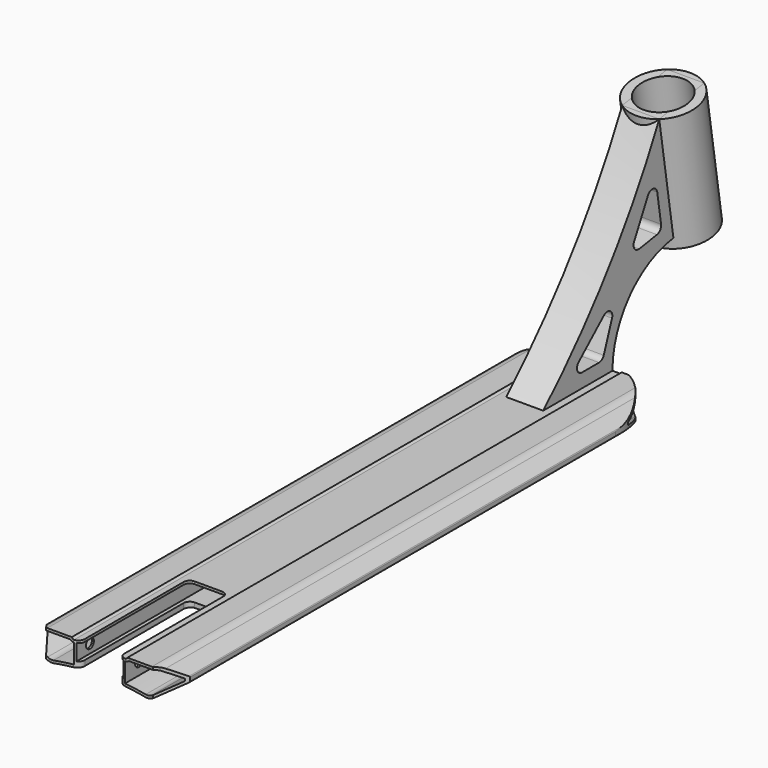
from build123d import *

# Parameters (mm, degrees)
F1_DEPTH       = 250
F2_W           = 38
F2_H           = 13
F3_DEPTH       = 250
F4_T1_DEPTH    = 500
F5_R           = 9
F6_R           = 1
F8_DEPTH       = 505
F10_DEPTH      = 118.9
F10_DEPTH_BACK = 563
F12_DEPTH      = 25
F12_DEPTH_BACK = 61.0714870032
F13_T1_DEPTH   = 2
F13_T6_DEPTH   = 32
F13_S7_R       = 200
F13_T8_DEPTH   = 18
F13_T13_DEPTH  = 32
F13_S14_R      = 200
F13_T15_DEPTH  = 18
F13_T20_DEPTH  = 64.2634824315
F13_T26_DEPTH  = 34.2634824315
F13_S27_R      = 200
F13_T28_DEPTH  = 19
F13_T32_DEPTH  = 34.2634824315
F13_S33_R      = 200
F13_T34_DEPTH  = 19
F13_T38_DEPTH  = 64.2634824315
F13_T41_DEPTH  = 62
F15_D          = 8
F15_DEPTH      = 50
F15_TIP        = 2.4034424761
F17_DEPTH      = 15
F18_R          = 27.5
F19_DEPTH      = 100
F21_D          = 40
F23_DEPTH      = 72.5010001
F24_R          = 5


# Not quite as in the source:
# - a fillet or chamfer that OpenCascade refuses, or shapes differently, is made with other operations: its cross-section is extruded or revolved along the edge and cut away or added
# - an extrude ends at something that could not be found from the text; its depth is read off the source's solid


with BuildPart() as f1:
    # F0 (on Front) → F1 (new body, symmetric)
    with BuildSketch(Plane.XZ):
        with BuildLine():
            Line((22.5, 59.7704869032), (0, 59.7704869032))
            Line((0, 59.7704869032), (-22.5, 59.7704869032))
            Line((-22.5, 59.7704869032), (-22.5, 61.0704869032))
            Line((-22.5, 61.0704869032), (-45.5824640741, 61.0704869032))
            Line((-45.5824640741, 61.0704869032), (-57.5, 51.0704869032))
            Line((-57.5, 51.0704869032), (-57.5, 47.0704869032))
            Line((-57.5, 47.0704869032), (-40.1794919243, 37.0704869032))
            ThreePointArc((-40.1794919243, 37.0704869032), (0, 41.1480317616), (40.1794919243, 37.0704869032))
            Line((40.1794919243, 37.0704869032), (57.5, 47.0704869032))
            Line((57.5, 47.0704869032), (57.5, 51.0704869032))
            Line((57.5, 51.0704869032), (45.5824640741, 61.0704869032))
            Line((45.5824640741, 61.0704869032), (22.5, 61.0704869032))
            Line((22.5, 61.0704869032), (22.5, 59.7704869032))
        make_face()
    extrude(amount=F1_DEPTH, both=True)

    # F2 (on Front) → F3 (cut, symmetric)
    with BuildSketch(Plane.XZ):
        with Locations((0, 51.2704869032)):
            Rectangle(F2_W, F2_H)
    extrude(amount=F3_DEPTH, both=True, mode=Mode.SUBTRACT)

    # F4: fillet of radius 2 on 2 edges, made by hand

    # F4_s2 → F4_t1 (join)
    with BuildSketch(Plane.XZ.offset(-250)):
        with BuildLine():
            ThreePointArc((22.5, 61.0704869032), (21.7666760256, 60.1273192307), (20.6265006005, 59.7704869032))
            Line((20.6265006005, 59.7704869032), (22.5, 59.7704869032))
            Line((22.5, 59.7704869032), (22.5, 61.0704869032))
        make_face()
        with BuildLine():
            ThreePointArc((-20.6265006005, 59.7704869032), (-21.7666760256, 60.1273192307), (-22.5, 61.0704869032))
            Line((-22.5, 61.0704869032), (-22.5, 59.7704869032))
            Line((-22.5, 59.7704869032), (-20.6265006005, 59.7704869032))
        make_face()
    extrude(amount=F4_T1_DEPTH)

    # F5
    f5_edges = [f1.edges().sort_by_distance(p)[0] for p in [
        (45.582464, 0, 61.070487),
        (-45.582464, 0, 61.070487),
        (-40.179492, 0, 37.070487),
        (40.179492, 0, 37.070487),
    ]]
    fillet(f5_edges, radius=F5_R)

    # F6
    f6_edges = [f1.edges().sort_by_distance(p)[0] for p in [
        (57.5, 0, 51.070487),
        (57.5, 0, 47.070487),
        (-57.5, 0, 51.070487),
        (-57.5, 0, 47.070487),
    ]]
    fillet(f6_edges, radius=F6_R)

    # F7 (on face) → F8 (cut)
    with BuildSketch(Plane.XZ.offset(250)):
        with BuildLine():
            ThreePointArc((20.6265006005, 42.0921719424), (28.9931861118, 41.0564987136), (37.3093701274, 39.6726168907))
            ThreePointArc((37.3093701274, 39.6726168907), (39.7790673433, 39.6518088424), (42.1022690923, 40.4900038955))
            Line((42.1022690923, 40.4900038955), (55.5, 48.2251874416))
            Line((55.5, 48.2251874416), (55.5, 50.1378715869))
            Line((55.5, 50.1378715869), (46.8062452335, 57.432798005))
            ThreePointArc((46.8062452335, 57.432798005), (44.7008729689, 58.6483352487), (42.3067319657, 59.0704869032))
            Line((42.3067319657, 59.0704869032), (23.5777715132, 59.0704869032))
            ThreePointArc((23.5777715132, 59.0704869032), (22.2389521501, 58.1098858596), (20.6265006005, 57.7704869032))
            Line((20.6265006005, 57.7704869032), (20.6265006005, 42.0921719424))
        make_face()
        with BuildLine():
            ThreePointArc((-37.3093701274, 39.6726168907), (-28.9931861118, 41.0564987136), (-20.6265006005, 42.0921719424))
            Line((-20.6265006005, 42.0921719424), (-20.6265006005, 57.7704869032))
            ThreePointArc((-20.6265006005, 57.7704869032), (-22.2389521501, 58.1098858596), (-23.5777715132, 59.0704869032))
            Line((-23.5777715132, 59.0704869032), (-42.3067319657, 59.0704869032))
            ThreePointArc((-42.3067319657, 59.0704869032), (-44.7008729689, 58.6483352487), (-46.8062452335, 57.432798005))
            Line((-46.8062452335, 57.432798005), (-55.5, 50.1378715869))
            Line((-55.5, 50.1378715869), (-55.5, 48.2251874416))
            Line((-55.5, 48.2251874416), (-42.1022690923, 40.4900038955))
            ThreePointArc((-42.1022690923, 40.4900038955), (-39.7790673433, 39.6518088424), (-37.3093701274, 39.6726168907))
        make_face()
    extrude(amount=-F8_DEPTH, mode=Mode.SUBTRACT)

    # F9 (on Top) → F10 (cut, two sides)
    with BuildSketch(Plane.XY) as f10_sk:
        with BuildLine():
            ThreePointArc((-57.5, 200), (0, 257.5), (57.5, 200))
            Line((57.5, 200), (57.5, 280))
            Line((57.5, 280), (-57.5, 280))
            Line((-57.5, 280), (-57.5, 200))
        make_face()
    extrude(amount=F10_DEPTH, mode=Mode.SUBTRACT)
    extrude(f10_sk.sketch, amount=-F10_DEPTH_BACK, mode=Mode.SUBTRACT)

    # F11 (on Top) → F12 (cut, two sides)
    with BuildSketch(Plane.XY) as f12_sk:
        Polygon((-68, -346), (68, -346), (68, -216), (43.2975540478, -250), (16, -250), (16, -140), (-16, -140), (-16, -250), (-43.2975540478, -250), (-68, -216), align=None)
    extrude(amount=-F12_DEPTH, mode=Mode.SUBTRACT)
    extrude(f12_sk.sketch, amount=F12_DEPTH_BACK, mode=Mode.SUBTRACT)

    # F13: fillet of radius 5 on 6 edges, made by hand

    # F13_s2 → F13_t1 (join)
    with BuildSketch(Plane.XY.offset(57.7704869032)):
        with BuildLine():
            ThreePointArc((-11, -140), (-14.5355339059, -141.4644660941), (-16, -145))
            Line((-16, -145), (-16.1, -145))
            Line((-16.1, -145), (-16.1, -139.9))
            Line((-16.1, -139.9), (-11, -139.9))
            Line((-11, -139.9), (-11, -140))
        make_face()
        with BuildLine():
            ThreePointArc((16, -145), (14.5355339059, -141.4644660941), (11, -140))
            Line((11, -140), (11, -139.9))
            Line((11, -139.9), (16.1, -139.9))
            Line((16.1, -139.9), (16.1, -145))
            Line((16.1, -145), (16, -145))
        make_face()
    extrude(amount=F13_T1_DEPTH)


with BuildPart() as f13_tool4:
    # F13_s5 → F13_t6 (new body)
    with BuildSketch(Plane.XY.offset(59.7704869032)):
        with BuildLine():
            ThreePointArc((-11, -140), (-14.5355339059, -141.4644660941), (-16, -145))
            Line((-16, -145), (-16.1, -145))
            Line((-16.1, -145), (-16.1, -139.9))
            Line((-16.1, -139.9), (-11, -139.9))
            Line((-11, -139.9), (-11, -140))
        make_face()
    extrude(amount=-F13_T6_DEPTH)

    # F13_s7 → F13_t8 (cut, symmetric)
    with BuildSketch(Plane.XZ.offset(142.4)):
        with Locations((0, -158.8519682384)):
            Circle(F13_S7_R)
    extrude(amount=F13_T8_DEPTH, both=True, mode=Mode.SUBTRACT)

    split(bisect_by=Plane.XY.offset(44.7704869032), keep=Keep.BOTTOM)


with BuildPart() as f1_1:
    add(f1.part)

    # F13_t3: union F13_tool4
    add(f13_tool4.part)


with BuildPart() as f13_tool11:
    # F13_s12 → F13_t13 (new body)
    with BuildSketch(Plane.XY.offset(27.7704869032)):
        with BuildLine():
            ThreePointArc((16, -145), (14.5355339059, -141.4644660941), (11, -140))
            Line((11, -140), (11, -139.9))
            Line((11, -139.9), (16.1, -139.9))
            Line((16.1, -139.9), (16.1, -145))
            Line((16.1, -145), (16, -145))
        make_face()
    extrude(amount=F13_T13_DEPTH)

    # F13_s14 → F13_t15 (cut, symmetric)
    with BuildSketch(Plane.XZ.offset(142.4)):
        with Locations((0, -158.8519682384)):
            Circle(F13_S14_R)
    extrude(amount=F13_T15_DEPTH, both=True, mode=Mode.SUBTRACT)

    split(bisect_by=Plane.XY.offset(44.7704869032), keep=Keep.BOTTOM)


with BuildPart() as f1_2:
    add(f1_1.part)

    # F13_t10: union F13_tool11
    add(f13_tool11.part)


with BuildPart() as f13_tool18:
    # F13_s19 → F13_t20 (new body)
    with BuildSketch(Plane.XY.offset(74.7704869032)):
        with BuildLine():
            ThreePointArc((-16, -145), (-14.5355339059, -141.4644660941), (-11, -140))
            Line((-11, -140), (-11, -139.9))
            Line((-11, -139.9), (-16.1, -139.9))
            Line((-16.1, -139.9), (-16.1, -145))
            Line((-16.1, -145), (-16, -145))
        make_face()
    extrude(amount=-F13_T20_DEPTH)

    split(bisect_by=Plane.XY.offset(57.7704869032), keep=Keep.TOP)

    split(bisect_by=Plane.XY.offset(59.7704869032), keep=Keep.BOTTOM)


with BuildPart() as f1_3:
    add(f1_2.part)

    # F13_t17: union F13_tool18
    add(f13_tool18.part)


with BuildPart() as f13_tool24:
    # F13_s25 → F13_t26 (new body)
    with BuildSketch(Plane.XY.offset(44.7704869032)):
        with BuildLine():
            ThreePointArc((-16, -145), (-14.5355339059, -141.4644660941), (-11, -140))
            Line((-11, -140), (-11, -139.9))
            Line((-11, -139.9), (-16.1, -139.9))
            Line((-16.1, -139.9), (-16.1, -145))
            Line((-16.1, -145), (-16, -145))
        make_face()
    extrude(amount=-F13_T26_DEPTH)

    # F13_s27 → F13_t28 (cut, symmetric)
    with BuildSketch(Plane.XZ.offset(142.4)):
        with Locations((0, -158.8519682384)):
            Circle(F13_S27_R)
    extrude(amount=F13_T28_DEPTH, both=True, mode=Mode.SUBTRACT)


with BuildPart() as f1_4:
    add(f1_3.part)

    # F13_t23: union F13_tool24
    add(f13_tool24.part)


with BuildPart() as f13_tool30:
    # F13_s31 → F13_t32 (new body)
    with BuildSketch(Plane.XY.offset(10.5070044716)):
        with BuildLine():
            ThreePointArc((16, -145), (14.5355339059, -141.4644660941), (11, -140))
            Line((11, -140), (11, -139.9))
            Line((11, -139.9), (16.1, -139.9))
            Line((16.1, -139.9), (16.1, -145))
            Line((16.1, -145), (16, -145))
        make_face()
    extrude(amount=F13_T32_DEPTH)

    # F13_s33 → F13_t34 (cut, symmetric)
    with BuildSketch(Plane.XZ.offset(142.4)):
        with Locations((0, -158.8519682384)):
            Circle(F13_S33_R)
    extrude(amount=F13_T34_DEPTH, both=True, mode=Mode.SUBTRACT)


with BuildPart() as f1_5:
    add(f1_4.part)

    # F13_t29: union F13_tool30
    add(f13_tool30.part)


with BuildPart() as f13_tool36:
    # F13_s37 → F13_t38 (new body)
    with BuildSketch(Plane.XY.offset(10.5070044716)):
        with BuildLine():
            ThreePointArc((16, -145), (14.5355339059, -141.4644660941), (11, -140))
            Line((11, -140), (11, -139.9))
            Line((11, -139.9), (16.1, -139.9))
            Line((16.1, -139.9), (16.1, -145))
            Line((16.1, -145), (16, -145))
        make_face()
    extrude(amount=F13_T38_DEPTH)

    split(bisect_by=Plane.XY.offset(57.7704869032), keep=Keep.TOP)

    split(bisect_by=Plane.XY.offset(59.7704869032), keep=Keep.BOTTOM)


with BuildPart() as f1_6:
    add(f1_5.part)

    # F13_t35: union F13_tool36
    add(f13_tool36.part)

    # F13_s42 → F13_t41 (cut)
    with BuildSketch(Plane.XY.offset(27.7704869032)):
        with BuildLine():
            ThreePointArc((-21, -250), (-17.4644660941, -248.5355339059), (-16, -245))
            Line((-16, -245), (-15.9, -245))
            Line((-15.9, -245), (-15.9, -250.1))
            Line((-15.9, -250.1), (-21, -250.1))
            Line((-21, -250.1), (-21, -250))
        make_face()
        with BuildLine():
            ThreePointArc((21, -250), (17.4644660941, -248.5355339059), (16, -245))
            Line((16, -245), (15.9, -245))
            Line((15.9, -245), (15.9, -250.1))
            Line((15.9, -250.1), (21, -250.1))
            Line((21, -250.1), (21, -250))
        make_face()
    extrude(amount=F13_T41_DEPTH, mode=Mode.SUBTRACT)

    # F15 (one way)
    with BuildSketch(Plane.YZ.offset(20.6265006005)):
        with Locations((-235.9860303046, 52.0921719424)):
            Circle(F15_D / 2)
    extrude(amount=-F15_DEPTH, mode=Mode.SUBTRACT)
    with Locations(Plane.YZ.offset(20.6265006005)):
        with Locations((-235.9860303046, 52.0921719424)):
            with Locations((0, 0, -(F15_DEPTH + F15_TIP / 2))):  # 118° drill point
                Cone(0, F15_D / 2, F15_TIP, mode=Mode.SUBTRACT)

    # F16 (on Right) → F17 (join, symmetric)
    with BuildSketch(Plane.YZ):
        with BuildLine():
            ThreePointArc((297.3819995028, 219.7704869032), (245.9666940414, 134.4327647562), (180, 59.7704869032))
            Line((180, 59.7704869032), (250, 59.7704869032))
            ThreePointArc((250, 59.7704869032), (267.6550746197, 106.2463815899), (311.7145367693, 129.2784080277))
            Line((311.7145367693, 129.2784080277), (313.0254460068, 121.0016528437))
            Line((313.0254460068, 121.0016528437), (358.4591096742, 128.1976382355))
            Line((358.4591096742, 128.1976382355), (342.8156631702, 226.966472295))
            Line((342.8156631702, 226.966472295), (297.3819995028, 219.7704869032))
        make_face()
    extrude(amount=F17_DEPTH, both=True)

    # F18 (on face) → F19 (join)
    with BuildSketch(Plane(origin=(0, -26.6789521342, 168.4442744471), x_dir=(1, 0, 0), z_dir=(0, -0.156434465, 0.9876883406))):
        with Locations((0, 351.1004121621)):
            Circle(F18_R)
    extrude(amount=-F19_DEPTH)

    # F21 (through all)
    with Locations(Plane(origin=(0, -26.6789521342, 168.4442744471), x_dir=(1, 0, 0), z_dir=(0, -0.156434465, 0.9876883406))):
        with Locations((0, 351.1004121621)):
            Hole(F21_D / 2)

    # F22 (on face) → F23 (cut, through all)
    with BuildSketch(Plane.YZ.offset(15)):
        Polygon((292.9320627918, 183.6294067652), (267.377898479, 134.021094092), (299.9716137186, 139.1834314384), align=None)
        Polygon((256.378660542, 116.0704869032), (206, 71.0704869032), (240, 71.0704869032), align=None)
    extrude(amount=-F23_DEPTH, mode=Mode.SUBTRACT)

    # F24
    f24_edges = [f1_6.edges().sort_by_distance(p)[0] for p in [
        (0, 299.971614, 139.183431),
        (0, 292.932063, 183.629407),
        (0, 267.377898, 134.021094),
        (0, 206, 71.070487),
        (0, 240, 71.070487),
        (0, 256.378661, 116.070487),
    ]]
    fillet(f24_edges, radius=F24_R)


solid = f1_6.part
